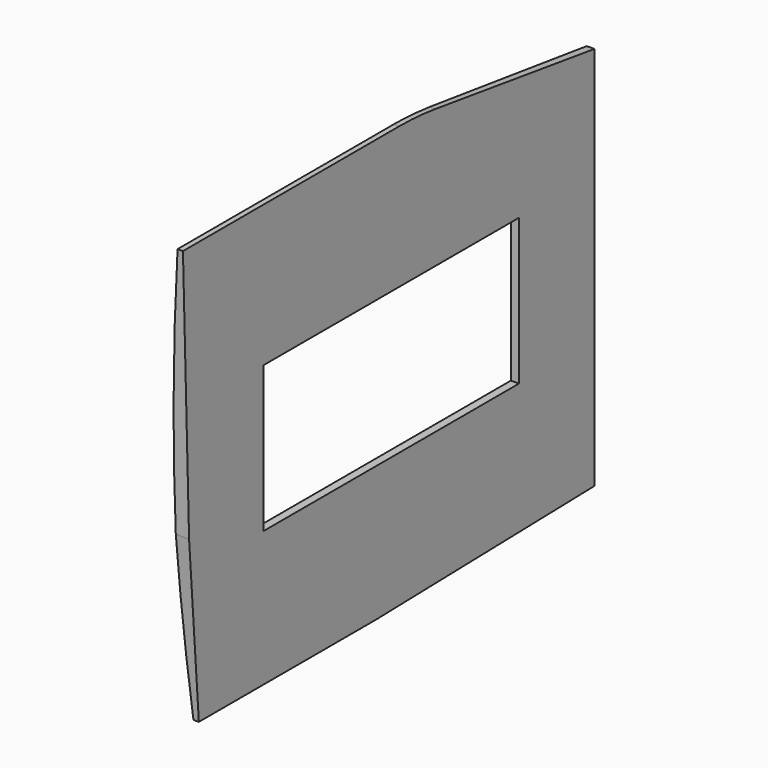
from build123d import *

# Parameters (mm, degrees)
F1_DEPTH      = 50
F2_W          = 67.5757344365
F2_H          = 156.2989021295
F3_DEPTH      = 250.3970603371
F3_DEPTH_BACK = 7.3495271517
F4_W          = 118
F4_H          = 54
F5_DEPTH      = 3.0593451962
F5_DEPTH_BACK = 2.001
F7_W          = 140
F7_H          = 75
F8_DEPTH      = 25
F9_W          = 87.5550785909
F9_H          = 196.2326095419
F10_DEPTH     = 5.0593451962


with BuildPart() as f1:
    # F0 (on Right) → F1 (new body, symmetric)
    with BuildSketch(Plane.YZ):
        with BuildLine():
            Line((-4.5147020681, 61.3411776654), (0, 0))
            Line((0, 0), (80, 0))
            ThreePointArc((80, 0), (81.4660401002, 0.0089556407), (82.9318613783, 0.0358212263))
            Line((82.9318613783, 0.0358212263), (182.9020103564, 2.4790390415))
            ThreePointArc((182.9020103564, 2.4790390415), (187.6095215539, 2.6866314133), (192.3052533926, 3.0788797612))
            Line((192.3052533926, 3.0788797612), (237.0668801629, 7.7045439166))
            ThreePointArc((237.0668801629, 7.7045439166), (244.0081250748, 10.8561399368), (247.6503203917, 17.5529938008))
            ThreePointArc((247.6503203917, 17.5529938008), (250.0657087208, 59.7730943442), (242.5639369549, 101.3915326986))
            ThreePointArc((242.5639369549, 101.3915326986), (226.8577665619, 127.0421650064), (200.677105552, 141.847965062))
            ThreePointArc((200.677105552, 141.847965062), (197.1231870334, 142.6835068064), (193.5250308066, 143.3013567969))
            Line((193.5250308066, 143.3013567969), (109.3522449635, 155.1310703785))
            ThreePointArc((109.3522449635, 155.1310703785), (101.0222496976, 156.0065881607), (92.6514728483, 156.2989021295))
            Line((92.6514728483, 156.2989021295), (-7.3485271517, 156.2989021295))
            Line((-7.3485271517, 156.2989021295), (-4.5147020681, 61.3411776654))
        make_face()
    extrude(amount=F1_DEPTH, both=True)

    # F2 (on Front) → F3 (cut, two sides)
    with BuildSketch(Plane.XZ) as f3_sk:
        with BuildLine():
            ThreePointArc((0, 0), (-3.0583450882, 78.1494510648), (0, 156.2989021295))
            Line((0, 156.2989021295), (-64.2212554812, 156.2989021295))
            Line((-64.2212554812, 156.2989021295), (-64.2212554812, 0))
            Line((-64.2212554812, 0), (0, 0))
        make_face()
        with Locations((35.7878672183, 78.1494510648)):
            Rectangle(F2_W, F2_H)
    extrude(amount=-F3_DEPTH, mode=Mode.SUBTRACT)
    extrude(f3_sk.sketch, amount=F3_DEPTH_BACK, mode=Mode.SUBTRACT)

    # F4 (on Right) → F5 (cut, two sides)
    with BuildSketch(Plane.YZ) as f5_sk:
        with Locations((89, 77)):
            Rectangle(F4_W, F4_H)
    extrude(amount=-F5_DEPTH, mode=Mode.SUBTRACT)
    extrude(f5_sk.sketch, amount=F5_DEPTH_BACK, mode=Mode.SUBTRACT)

    # F7 (on offset) → F8 (cut)
    with BuildSketch(Plane.YZ.offset(-1)):
        with Locations((89, 77)):
            Rectangle(F7_W, F7_H)
    extrude(amount=-F8_DEPTH, mode=Mode.SUBTRACT)

    # F9 (on face) → F10 (cut, through all)
    with BuildSketch(Plane.YZ.offset(2)):
        with Locations((226.6795496519, 100.5953438125)):
            Rectangle(F9_W, F9_H)
    extrude(amount=-F10_DEPTH, mode=Mode.SUBTRACT)


solid = f1.part
